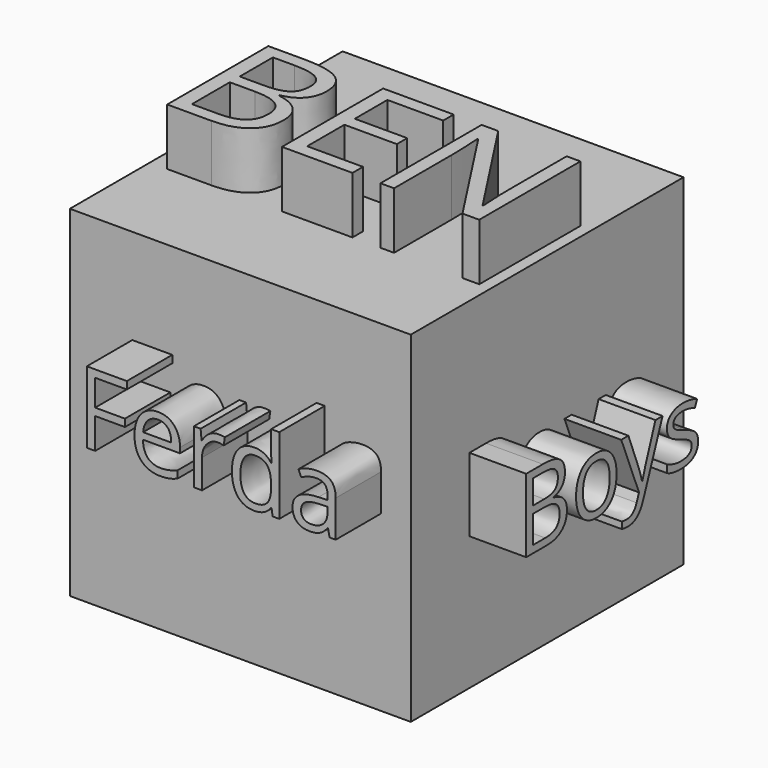
from build123d import *

# Parameters (mm, degrees)
F0_W         = 76.2
F0_H         = 76.2
F1_DEPTH     = 76.2
F2_TEXT_SIZE = 39.5908426693
F3_DEPTH     = 12.7
F4_TEXT_SIZE = 22.4707738703
F5_DEPTH     = 12.7
F6_TEXT_SIZE = 22.9974332291
F7_DEPTH     = 12.7


# Not quite as in the source:
# - Text() gives the source's letters only with a copy of the font that has no kerning and outlines rounded to 1/6400 em; it was checked with that copy


with BuildPart() as f1:
    # F0 (on Front) → F1 (new body)
    with BuildSketch(Plane.XZ):
        with Locations((-3.2231509686, 10.8602594644)):
            Rectangle(F0_W, F0_H)
    extrude(amount=F1_DEPTH)

    # F2 (on face) → F3 (join)
    with BuildSketch(Plane.XY.offset(48.9602594644)):
        with Locations((-41.3231509686, -53.8593260374)):
            Text('BEN', F2_TEXT_SIZE, font='Open Sans', text_align=(TextAlign.LEFT, TextAlign.BOTTOM))
    extrude(amount=F3_DEPTH)

    # F4 (on face) → F5 (join)
    with BuildSketch(Plane.XZ.offset(76.2)):
        with Locations((-29.5771546662, 11.6156386212)):
            Text('Ferda', F4_TEXT_SIZE, font='Open Sans', text_align=(TextAlign.LEFT, TextAlign.BOTTOM))
    extrude(amount=F5_DEPTH)

    # F6 (on face) → F7 (join)
    with BuildSketch(Plane.YZ.offset(34.8768490314)):
        with Locations((-62.0825365186, 2.6413740125)):
            Text('Boys', F6_TEXT_SIZE, font='Open Sans', text_align=(TextAlign.LEFT, TextAlign.BOTTOM))
    extrude(amount=F7_DEPTH)


solid = f1.part
